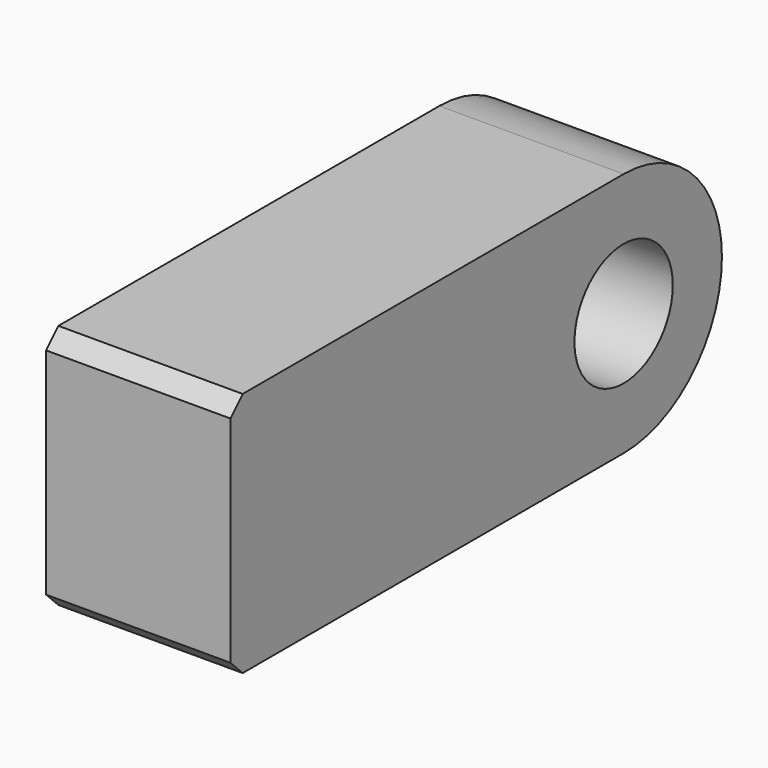
from build123d import *

# Parameters (mm, degrees)
F0_W     = 63.5
F0_H     = 25.4
F1_DEPTH = 19.05
F2_R     = 6.35
F3_DEPTH = 25.4
F4_R     = 12.69999
F5_SIZE  = 1.5875


# Not quite as in the source:
# - a fillet or chamfer is up to 0.001 mm smaller than in the source, because OpenCascade refuses the exact size


with BuildPart() as f1:
    # F0 (on Right) → F1 (new body)
    with BuildSketch(Plane.YZ):
        Rectangle(F0_W, F0_H)
    extrude(amount=F1_DEPTH)

    # F2 (on face) → F3 (cut)
    with BuildSketch(Plane.YZ.offset(19.05)):
        with Locations((19.05, 0)):
            Circle(F2_R)
    extrude(amount=-F3_DEPTH, mode=Mode.SUBTRACT)

    # F4 (radius 12.7 in the source; OpenCascade refuses exactly that, so slightly less here)
    f4_edges = [f1.edges().sort_by_distance(p)[0] for p in [
        (9.525, 31.75, 12.7),
        (9.525, 31.75, -12.7),
    ]]
    fillet(f4_edges, radius=F4_R)

    # F5
    f5_edges = [f1.edges().sort_by_distance(p)[0] for p in [
        (9.525, -31.75, 12.7),
        (9.525, -31.75, -12.7),
    ]]
    chamfer(f5_edges, length=F5_SIZE)


solid = f1.part
